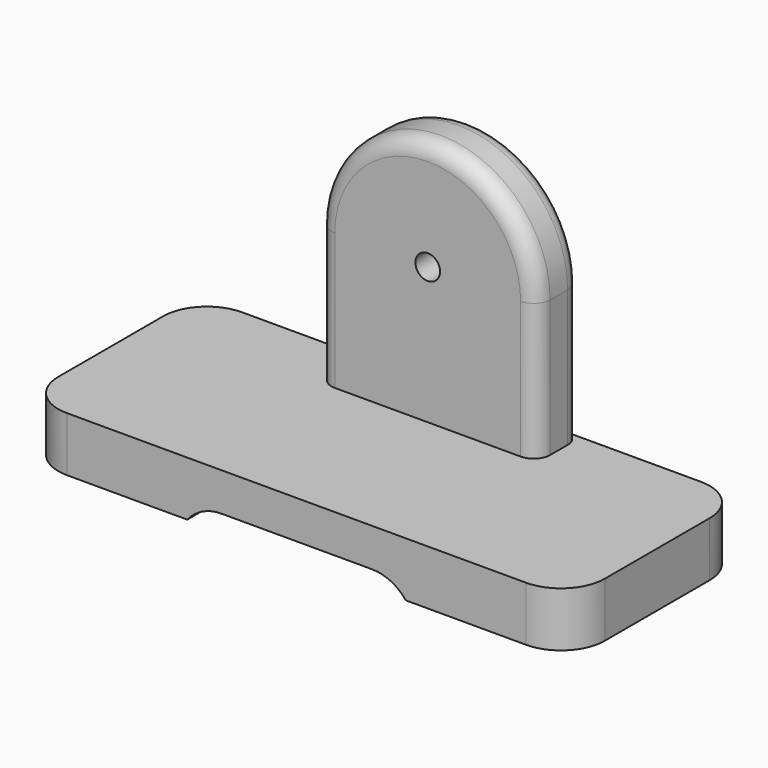
from build123d import *

# Parameters (mm, degrees)
F0_W          = 100
F0_H          = 40
F1_DEPTH      = 10
F4_DEPTH      = 10
F5_W          = 40
F5_H          = 3
F6_DEPTH      = 40.001
F7_R          = 2.25
F8_DEPTH      = 40.001
F9_R          = 4.5
F10_DEPTH     = 5.7
F11_T1_DEPTH  = 40
F11_T3_DEPTH  = 40
F11_T5_DEPTH  = 50
F11_T7_DEPTH  = 50
F11_T9_DEPTH  = 50
F11_T11_DEPTH = 50
F12_R         = 3


# Not quite as in the source:
# - a fillet or chamfer that OpenCascade refuses, or shapes differently, is made with other operations: its cross-section is extruded or revolved along the edge and cut away or added


with BuildPart() as f1:
    # F0 (on Top) → F1 (new body)
    with BuildSketch(Plane.XY):
        with Locations((50, 20)):
            Rectangle(F0_W, F0_H)
    extrude(amount=F1_DEPTH)

    # F3 (on face) → F4 (join)
    with BuildSketch(Plane(origin=(0, 40, 0), x_dir=(-1, 0, 0), z_dir=(0, 1, 0))):
        with BuildLine():
            Line((-70, 35), (-70, 0))
            Line((-70, 0), (-30, 0))
            Line((-30, 0), (-30, 35))
            ThreePointArc((-30, 35), (-50, 55), (-70, 35))
        make_face()
    extrude(amount=-F4_DEPTH)

    # F5 (on face) → F6 (cut, through all)
    with BuildSketch(Plane(origin=(0, 40, 0), x_dir=(-1, 0, 0), z_dir=(0, 1, 0))):
        with Locations((-50, 1.5)):
            Rectangle(F5_W, F5_H)
    extrude(amount=-F6_DEPTH, mode=Mode.SUBTRACT)

    # F7 (on face) → F8 (cut, through all)
    with BuildSketch(Plane(origin=(0, 40, 0), x_dir=(-1, 0, 0), z_dir=(0, 1, 0))):
        with Locations((-50, 35)):
            Circle(F7_R)
    extrude(amount=-F8_DEPTH, mode=Mode.SUBTRACT)

    # F9 (on face) → F10 (cut)
    with BuildSketch(Plane(origin=(0, 40, 0), x_dir=(-1, 0, 0), z_dir=(0, 1, 0))):
        with Locations((-50, 35)):
            Circle(F9_R)
    extrude(amount=-F10_DEPTH, mode=Mode.SUBTRACT)

    # F11: fillet of radius 8 on 6 edges, made by hand

    # F11_s2 → F11_t1 (join)
    with BuildSketch(Plane.XZ.offset(-40)):
        with BuildLine():
            ThreePointArc((70, 0), (67.2191036167, 2.2111025509), (63.7550020016, 3))
            Line((63.7550020016, 3), (70, 3))
            Line((70, 3), (70, 0))
        make_face()
    extrude(amount=F11_T1_DEPTH)

    # F11_s4 → F11_t3 (join)
    with BuildSketch(Plane.XZ.offset(-40)):
        with BuildLine():
            ThreePointArc((36.2449979984, 3), (32.7808963833, 2.2111025509), (30, 0))
            Line((30, 0), (30, 3))
            Line((30, 3), (36.2449979984, 3))
        make_face()
    extrude(amount=F11_T3_DEPTH)

    # F11_s6 → F11_t5 (cut)
    with BuildSketch(Plane.XY.offset(-20)):
        with BuildLine():
            ThreePointArc((0, 32), (2.3431457505, 37.6568542495), (8, 40))
            Line((8, 40), (0, 40))
            Line((0, 40), (0, 32))
        make_face()
    extrude(amount=F11_T5_DEPTH, mode=Mode.SUBTRACT)

    # F11_s8 → F11_t7 (cut)
    with BuildSketch(Plane.XY.offset(-20)):
        with BuildLine():
            ThreePointArc((0, 8), (2.3431457505, 2.3431457505), (8, 0))
            Line((8, 0), (0, 0))
            Line((0, 0), (0, 8))
        make_face()
    extrude(amount=F11_T7_DEPTH, mode=Mode.SUBTRACT)

    # F11_s10 → F11_t9 (cut)
    with BuildSketch(Plane.XY.offset(-20)):
        with BuildLine():
            ThreePointArc((92, 40), (97.6568542495, 37.6568542495), (100, 32))
            Line((100, 32), (100, 40))
            Line((100, 40), (92, 40))
        make_face()
    extrude(amount=F11_T9_DEPTH, mode=Mode.SUBTRACT)

    # F11_s12 → F11_t11 (cut)
    with BuildSketch(Plane.XY.offset(-20)):
        with BuildLine():
            ThreePointArc((92, 0), (97.6568542495, 2.3431457505), (100, 8))
            Line((100, 8), (100, 0))
            Line((100, 0), (92, 0))
        make_face()
    extrude(amount=F11_T11_DEPTH, mode=Mode.SUBTRACT)

    # F12
    f12_edges = [f1.edges().sort_by_distance(p)[0] for p in [
        (50, 40, 55),
        (50, 30, 55),
        (30, 40, 22.5),
        (70, 40, 22.5),
        (30, 30, 22.5),
        (70, 30, 22.5),
    ]]
    fillet(f12_edges, radius=F12_R)


solid = f1.part
